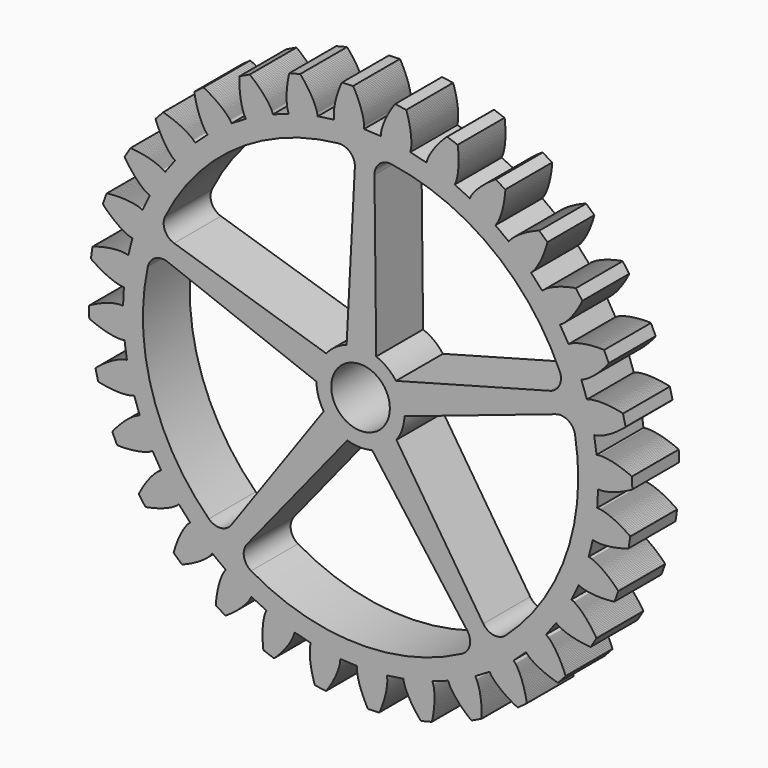
from build123d import *

# Parameters (mm, degrees)
F0_R     = 4
F1_DEPTH = 8


# Not quite as in the source:
# - ends of sketch curves that miss each other by under 0.0002 mm in the source are joined


with BuildPart() as f1:
    # F0 (on Front) → F1 (new body)
    with BuildSketch(Plane.XZ):
        Polygon((-32.30495, 2.758791), (-32.418904, 0.483381), (-32.827953, 0.489421), (-32.836156, 0.489353), (-32.848265, 0.489121), (-32.864272, 0.488639), (-32.884176, 0.487826), (-32.90797, 0.486592), (-32.93565, 0.484856), (-32.967203, 0.482529), (-33.002622, 0.47953), (-33.041894, 0.475776), (-33.085007, 0.471178), (-33.131944, 0.465651), (-33.182695, 0.459117), (-33.237238, 0.45149), (-33.29556, 0.442681), (-33.357637, 0.432614), (-33.423449, 0.421205), (-33.492973, 0.408367), (-33.566185, 0.394022), (-33.643063, 0.378087), (-33.723579, 0.36048), (-33.807704, 0.341119), (-33.89541, 0.319922), (-33.986665, 0.296816), (-34.081439, 0.271712), (-34.179699, 0.244537), (-34.281407, 0.215206), (-34.386532, 0.183647), (-34.495036, 0.149779), (-34.60688, 0.113524), (-34.722023, 0.07481), (-34.840427, 0.033554), (-34.962046, -0.010314), (-35.086841, -0.056873), (-35.214765, -0.106196), (-35.345772, -0.158355), (-35.479815, -0.213426), (-35.616844, -0.271479), (-35.756814, -0.332584), (-35.899674, -0.396816), (-36.045365, -0.464242), (-36.19384, -0.534931), (-36.345044, -0.608957), (-36.498922, -0.686378), (-36.655413, -0.767272), (-36.814466, -0.851694), (-36.976019, -0.939718), (-37.102372, -1.03036), (-37.029669, -2.539949), (-36.895187, -2.618028), (-36.725926, -2.69012), (-36.559495, -2.758869), (-36.395953, -2.824345), (-36.235347, -2.886624), (-36.077731, -2.945775), (-35.923148, -3.001868), (-35.771652, -3.05498), (-35.623283, -3.105186), (-35.478088, -3.152558), (-35.336111, -3.197173), (-35.197396, -3.239109), (-35.061983, -3.278438), (-34.929912, -3.315237), (-34.801221, -3.349589), (-34.67595, -3.381567), (-34.55413, -3.411253), (-34.435797, -3.438723), (-34.320987, -3.464063), (-34.209733, -3.487346), (-34.102062, -3.508656), (-33.998002, -3.528075), (-33.897586, -3.545683), (-33.800839, -3.56156), (-33.707785, -3.575794), (-33.618449, -3.588462), (-33.532853, -3.599649), (-33.45102, -3.609438), (-33.372967, -3.617912), (-33.298711, -3.625154), (-33.228277, -3.631252), (-33.161672, -3.636284), (-33.098917, -3.640337), (-33.040018, -3.643499), (-32.984994, -3.645852), (-32.93385, -3.647479), (-32.886599, -3.648479), (-32.843243, -3.648928), (-32.80379, -3.648891), (-32.76825, -3.648471), (-32.736619, -3.647754), (-32.708902, -3.646824), (-32.685097, -3.645764), (-32.665206, -3.644662), (-32.649229, -3.643603), (-32.637155, -3.64267), (-32.628982, -3.64195), (-32.222407, -3.596628), (-31.890287, -5.850547), (-32.292656, -5.924424), (-32.30069, -5.926093), (-32.312516, -5.928684), (-32.328121, -5.932277), (-32.347486, -5.93696), (-32.370583, -5.94281), (-32.39739, -5.949914), (-32.427885, -5.958352), (-32.462036, -5.968202), (-32.499823, -5.979548), (-32.54121, -5.992468), (-32.586169, -6.007045), (-32.634668, -6.023353), (-32.686676, -6.041477), (-32.742158, -6.061491), (-32.801078, -6.083474), (-32.8634, -6.107507), (-32.929084, -6.13366), (-32.998093, -6.162015), (-33.070382, -6.192642), (-33.145916, -6.225619), (-33.224646, -6.261018), (-33.306532, -6.298915), (-33.391525, -6.339385), (-33.479581, -6.382493), (-33.570651, -6.428317), (-33.664684, -6.476926), (-33.761633, -6.528388), (-33.861445, -6.582774), (-33.964066, -6.640148), (-34.069445, -6.700586), (-34.177523, -6.764147), (-34.288249, -6.830899), (-34.40156, -6.900911), (-34.517406, -6.974242), (-34.635719, -7.050959), (-34.756442, -7.131121), (-34.879514, -7.21479), (-35.004876, -7.30203), (-35.132456, -7.392896), (-35.262195, -7.48745), (-35.394027, -7.585747), (-35.527884, -7.687849), (-35.663698, -7.793802), (-35.801404, -7.903672), (-35.940929, -8.017503), (-36.082204, -8.13535), (-36.188447, -8.248902), (-35.822632, -9.7153), (-35.675507, -9.765645), (-35.495432, -9.803327), (-35.318789, -9.838286), (-35.145615, -9.870601), (-34.975945, -9.90035), (-34.809816, -9.927615), (-34.64726, -9.952475), (-34.488312, -9.975011), (-34.332999, -9.995305), (-34.181354, -10.013442), (-34.0334, -10.0295), (-33.889169, -10.043566), (-33.748687, -10.055723), (-33.611973, -10.066051), (-33.479056, -10.074633), (-33.349949, -10.081559), (-33.224681, -10.086909), (-33.103262, -10.090766), (-32.985716, -10.09322), (-32.872055, -10.094351), (-32.762296, -10.094245), (-32.656447, -10.09299), (-32.554525, -10.090671), (-32.456539, -10.08737), (-32.362497, -10.083175), (-32.272405, -10.07817), (-32.186273, -10.072442), (-32.1041, -10.066078), (-32.025893, -10.059164), (-31.951655, -10.051781), (-31.881384, -10.044018), (-31.815079, -10.03596), (-31.752737, -10.027696), (-31.694353, -10.019304), (-31.639928, -10.010875), (-31.589447, -10.002496), (-31.542909, -9.994245), (-31.500305, -9.986214), (-31.461619, -9.978481), (-31.426839, -9.971136), (-31.395958, -9.964262), (-31.368954, -9.957941), (-31.345814, -9.952259), (-31.32652, -9.947296), (-31.311054, -9.943141), (-31.299397, -9.939873), (-31.291522, -9.937573), (-30.901601, -9.8138), (-30.136143, -11.959618), (-30.516371, -12.110574), (-30.523923, -12.113776), (-30.535017, -12.118625), (-30.549621, -12.125193), (-30.567698, -12.133564), (-30.589213, -12.14381), (-30.614117, -12.156006), (-30.64238, -12.170229), (-30.673955, -12.186554), (-30.708799, -12.205051), (-30.74687, -12.2258), (-30.788123, -12.248866), (-30.832511, -12.274325), (-30.879984, -12.302247), (-30.930496, -12.332701), (-30.983994, -12.365758), (-31.040427, -12.401483), (-31.099748, -12.439948), (-31.161897, -12.481222), (-31.226825, -12.525362), (-31.294475, -12.572442), (-31.364787, -12.622522), (-31.437703, -12.675668), (-31.513172, -12.731937), (-31.591124, -12.791399), (-31.671503, -12.854109), (-31.754247, -12.920128), (-31.839292, -12.989513), (-31.926575, -13.062327), (-32.016033, -13.138622), (-32.107594, -13.218453), (-32.201197, -13.30188), (-32.296773, -13.388952), (-32.394248, -13.479723), (-32.493562, -13.574246), (-32.594635, -13.672569), (-32.6974, -13.774741), (-32.801785, -13.880817), (-32.907717, -13.990836), (-33.015119, -14.104845), (-33.123918, -14.222894), (-33.234039, -14.345022), (-33.345407, -14.471274), (-33.457941, -14.601692), (-33.571567, -14.736312), (-33.686202, -14.875178), (-33.801772, -15.018324), (-33.883821, -15.150418), (-33.238955, -16.517272), (-33.084833, -16.537945), (-32.900866, -16.539774), (-32.720798, -16.539603), (-32.544647, -16.53751), (-32.372435, -16.533586), (-32.20418, -16.527916), (-32.039896, -16.520585), (-31.879605, -16.511678), (-31.72332, -16.501284), (-31.571049, -16.489487), (-31.422807, -16.476375), (-31.278602, -16.462033), (-31.138447, -16.446548), (-31.002345, -16.430006), (-30.870306, -16.412493), (-30.742332, -16.394097), (-30.618423, -16.374903), (-30.498586, -16.355001), (-30.38282, -16.334474), (-30.271124, -16.313412), (-30.163492, -16.291896), (-30.059923, -16.270015), (-29.960415, -16.247854), (-29.864955, -16.225501), (-29.773535, -16.203039), (-29.686154, -16.180556), (-29.602792, -16.158135), (-29.523439, -16.135863), (-29.448085, -16.11382), (-29.376712, -16.092097), (-29.309304, -16.070774), (-29.245845, -16.049936), (-29.186314, -16.029668), (-29.130691, -16.010049), (-29.078953, -15.991165), (-29.03108, -15.973095), (-28.987048, -15.955927), (-28.946828, -15.939737), (-28.910393, -15.924605), (-28.877716, -15.910618), (-28.848768, -15.89785), (-28.823514, -15.886383), (-28.80193, -15.876295), (-28.783973, -15.867664), (-28.769616, -15.860571), (-28.758821, -15.855088), (-28.751545, -15.851299), (-28.393263, -15.653834), (-27.223886, -17.609087), (-27.567356, -17.831322), (-27.574136, -17.835937), (-27.584075, -17.842854), (-27.597118, -17.852148), (-27.613215, -17.863883), (-27.632313, -17.878128), (-27.654361, -17.894952), (-27.679305, -17.914416), (-27.70709, -17.936585), (-27.737657, -17.961527), (-27.77095, -17.989303), (-27.806909, -18.019975), (-27.845476, -18.053601), (-27.886588, -18.090248), (-27.930189, -18.129971), (-27.976209, -18.17283), (-28.024591, -18.218881), (-28.075266, -18.26818), (-28.128171, -18.320783), (-28.183239, -18.376743), (-28.240401, -18.436115), (-28.299594, -18.498951), (-28.360742, -18.565299), (-28.42378, -18.635212), (-28.488635, -18.70874), (-28.555237, -18.785927), (-28.62351, -18.866819), (-28.693388, -18.951464), (-28.764789, -19.039905), (-28.83764, -19.132186), (-28.911869, -19.228348), (-28.987398, -19.328431), (-29.064148, -19.432475), (-29.142046, -19.54052), (-29.221006, -19.652599), (-29.300956, -19.768753), (-29.381814, -19.889011), (-29.463499, -20.01341), (-29.545931, -20.141983), (-29.629028, -20.274756), (-29.712707, -20.411761), (-29.796887, -20.553027), (-29.881482, -20.698581), (-29.966413, -20.848443), (-30.051592, -21.002645), (-30.136934, -21.161207), (-30.222355, -21.32415), (-30.277059, -21.469714), (-29.377922, -22.684498), (-29.22273, -22.674706), (-29.041943, -22.64061), (-28.865365, -22.60531), (-28.693007, -22.568894), (-28.524871, -22.531448), (-28.360953, -22.493061), (-28.20126, -22.453822), (-28.045785, -22.413816), (-27.894528, -22.373128), (-27.747484, -22.331853), (-27.604648, -22.29007), (-27.466014, -22.247871), (-27.331572, -22.20534), (-27.201315, -22.162564), (-27.075228, -22.11963), (-26.9533, -22.076622), (-26.835519, -22.033623), (-26.721866, -21.990724), (-26.61233, -21.948009), (-26.506888, -21.905557), (-26.405523, -21.863457), (-26.308213, -21.82179), (-26.21494, -21.780644), (-26.125674, -21.740096), (-26.040395, -21.700233), (-25.959078, -21.661132), (-25.88169, -21.62288), (-25.808211, -21.585555), (-25.738602, -21.549234), (-25.672841, -21.514006), (-25.610887, -21.479942), (-25.552712, -21.447122), (-25.498278, -21.415629), (-25.447552, -21.385538), (-25.400494, -21.356922), (-25.357066, -21.32986), (-25.317228, -21.304431), (-25.280937, -21.280705), (-25.248154, -21.258758), (-25.218835, -21.238662), (-25.192934, -21.220493), (-25.170404, -21.204318), (-25.151203, -21.190215), (-25.135277, -21.178245), (-25.122577, -21.168488), (-25.113059, -21.161004), (-25.106664, -21.155869), (-24.793788, -20.892301), (-23.265429, -22.581851), (-23.558942, -22.866824), (-23.564695, -22.872669), (-23.573089, -22.881398), (-23.584069, -22.893055), (-23.597569, -22.907707), (-23.613521, -22.925402), (-23.631866, -22.946202), (-23.652534, -22.970158), (-23.675457, -22.997323), (-23.700571, -23.02775), (-23.727804, -23.061486), (-23.757089, -23.098585), (-23.788353, -23.13909), (-23.82153, -23.183052), (-23.85654, -23.230518), (-23.893317, -23.281533), (-23.931785, -23.336137), (-23.971869, -23.394374), (-24.013495, -23.456287), (-24.056588, -23.521918), (-24.101067, -23.591302), (-24.146864, -23.664475), (-24.193893, -23.741479), (-24.242081, -23.822346), (-24.291345, -23.907112), (-24.341608, -23.995809), (-24.392792, -24.088466), (-24.444808, -24.18512), (-24.497585, -24.28579), (-24.551034, -24.390509), (-24.605076, -24.499307), (-24.65963, -24.612201), (-24.714606, -24.729219), (-24.769929, -24.850385), (-24.825507, -24.975717), (-24.881259, -25.105235), (-24.937103, -25.238958), (-24.992948, -25.376903), (-25.048715, -25.519087), (-25.10431, -25.665518), (-25.159654, -25.816218), (-25.214655, -25.97119), (-25.269233, -26.13045), (-25.323291, -26.294005), (-25.376749, -26.46186), (-25.429521, -26.634026), (-25.481512, -26.8105), (-25.506763, -26.963938), (-24.387916, -27.97997), (-24.237611, -27.94009), (-24.066949, -27.871379), (-23.900654, -27.802308), (-23.738711, -27.732966), (-23.581112, -27.663438), (-23.427831, -27.59381), (-23.278861, -27.52417), (-23.134179, -27.4546), (-22.993768, -27.385189), (-22.857601, -27.316019), (-22.725662, -27.247173), (-22.597924, -27.178739), (-22.474363, -27.110797), (-22.354951, -27.043431), (-22.239666, -26.976721), (-22.12847, -26.910753), (-22.02134, -26.845605), (-21.918243, -26.781356), (-21.819144, -26.71809), (-21.724007, -26.655884), (-21.632804, -26.594819), (-21.545495, -26.53497), (-21.462037, -26.476416), (-21.382399, -26.419233), (-21.306535, -26.363497), (-21.234409, -26.309284), (-21.165972, -26.256671), (-21.101186, -26.205725), (-21.040002, -26.156525), (-20.982376, -26.109144), (-20.928257, -26.063647), (-20.877603, -26.02011), (-20.830359, -25.978601), (-20.786478, -25.939191), (-20.745907, -25.901946), (-20.708593, -25.866932), (-20.67448, -25.834219), (-20.643518, -25.803869), (-20.615647, -25.775946), (-20.590811, -25.75052), (-20.568951, -25.727643), (-20.550012, -25.707386), (-20.533927, -25.689808), (-20.520643, -25.674962), (-20.510094, -25.662915), (-20.502214, -25.653717), (-20.496945, -25.647432), (-20.2415, -25.32789), (-18.412894, -26.686808), (-18.645173, -27.023566), (-18.649674, -27.030423), (-18.656207, -27.04062), (-18.664699, -27.054194), (-18.67508, -27.071199), (-18.687275, -27.091669), (-18.701209, -27.115646), (-18.716804, -27.143176), (-18.733988, -27.174291), (-18.752685, -27.209029), (-18.772815, -27.24743), (-18.7943, -27.289529), (-18.817059, -27.335356), (-18.841021, -27.384948), (-18.8661, -27.438333), (-18.892216, -27.495541), (-18.919294, -27.556599), (-18.947244, -27.621539), (-18.975994, -27.690385), (-19.005453, -27.763159), (-19.035545, -27.839885), (-19.066184, -27.920588), (-19.097289, -28.005287), (-19.128771, -28.094003), (-19.160552, -28.186752), (-19.192545, -28.28355), (-19.224667, -28.384411), (-19.25683, -28.489353), (-19.288953, -28.598389), (-19.320947, -28.711524), (-19.352724, -28.82877), (-19.384205, -28.950141), (-19.415295, -29.075635), (-19.445914, -29.205266), (-19.475975, -29.339033), (-19.505391, -29.476939), (-19.534072, -29.618986), (-19.561934, -29.765176), (-19.588888, -29.915507), (-19.614849, -30.069972), (-19.639728, -30.228571), (-19.663441, -30.391298), (-19.685896, -30.558144), (-19.70701, -30.729102), (-19.726694, -30.904161), (-19.744865, -31.083312), (-19.761428, -31.266541), (-19.756262, -31.421959), (-18.46069, -32.200188), (-18.321056, -32.131751), (-18.16708, -32.031066), (-18.017455, -31.93088), (-17.872152, -31.831278), (-17.731143, -31.732338), (-17.594393, -31.634148), (-17.461871, -31.536782), (-17.333542, -31.440323), (-17.209367, -31.344851), (-17.089313, -31.250447), (-16.97334, -31.157184), (-16.861408, -31.065144), (-16.753475, -30.974402), (-16.649502, -30.885034), (-16.549442, -30.797115), (-16.453257, -30.710721), (-16.360895, -30.625923), (-16.272311, -30.542798), (-16.187458, -30.461413), (-16.106287, -30.381843), (-16.02875, -30.304158), (-15.954794, -30.228427), (-15.884365, -30.154717), (-15.81741, -30.083094), (-15.75388, -30.01363), (-15.693714, -29.946387), (-15.636858, -29.881433), (-15.583254, -29.818827), (-15.532843, -29.758637), (-15.485567, -29.700923), (-15.441368, -29.645744), (-15.400179, -29.593159), (-15.361942, -29.543233), (-15.326591, -29.496018), (-15.294066, -29.451572), (-15.264301, -29.409954), (-15.237226, -29.371213), (-15.212778, -29.335405), (-15.190891, -29.302584), (-15.171492, -29.272796), (-15.154514, -29.246099), (-15.139892, -29.222535), (-15.127548, -29.202156), (-15.117414, -29.185004), (-15.109415, -29.171127), (-15.103483, -29.160574), (-15.099544, -29.153378), (-14.911346, -28.790142), (-12.852764, -29.766205), (-13.014881, -30.141808), (-13.017955, -30.149413), (-13.022375, -30.160687), (-13.028058, -30.175659), (-13.03492, -30.19436), (-13.042887, -30.216815), (-13.051876, -30.243051), (-13.061802, -30.273096), (-13.072586, -30.306963), (-13.084143, -30.344683), (-13.096394, -30.386274), (-13.109254, -30.431754), (-13.122636, -30.481144), (-13.136464, -30.534454), (-13.150645, -30.591705), (-13.165101, -30.652909), (-13.179744, -30.718077), (-13.194489, -30.787223), (-13.209254, -30.860355), (-13.223951, -30.937477), (-13.238495, -31.0186), (-13.2528, -31.103733), (-13.266782, -31.19287), (-13.280355, -31.286025), (-13.293431, -31.383191), (-13.305926, -31.48437), (-13.317752, -31.589562), (-13.328824, -31.698762), (-13.339057, -31.811966), (-13.348364, -31.929171), (-13.356659, -32.050363), (-13.363855, -32.175542), (-13.369865, -32.304692), (-13.374608, -32.437804), (-13.377994, -32.574867), (-13.379933, -32.715862), (-13.380351, -32.860774), (-13.379157, -33.009592), (-13.376265, -33.16229), (-13.371594, -33.318853), (-13.365054, -33.47926), (-13.356563, -33.643486), (-13.346038, -33.811505), (-13.333396, -33.9833), (-13.318549, -34.158835), (-13.301415, -34.338089), (-13.281916, -34.521027), (-13.246527, -34.672451), (-11.824027, -35.182975), (-11.700429, -35.08861), (-11.56905, -34.95982), (-11.441847, -34.832369), (-11.318766, -34.706334), (-11.199769, -34.581787), (-11.084804, -34.458802), (-10.973824, -34.337454), (-10.866776, -34.217812), (-10.763617, -34.09995), (-10.664284, -33.983937), (-10.568734, -33.869843), (-10.476908, -33.757734), (-10.388755, -33.647679), (-10.304213, -33.539743), (-10.223228, -33.433993), (-10.145746, -33.330494), (-10.071701, -33.229308), (-10.001035, -33.130496), (-9.933692, -33.034124), (-9.869605, -32.940248), (-9.808713, -32.848928), (-9.75095, -32.760221), (-9.696255, -32.674187), (-9.644563, -32.590879), (-9.595804, -32.510357), (-9.549911, -32.432669), (-9.506818, -32.35787), (-9.466459, -32.286011), (-9.428761, -32.217141), (-9.393653, -32.151313), (-9.361068, -32.088571), (-9.330927, -32.028963), (-9.303165, -31.972533), (-9.277708, -31.919331), (-9.254479, -31.869394), (-9.233401, -31.822766), (-9.214407, -31.77949), (-9.197416, -31.7396), (-9.182349, -31.703138), (-9.169135, -31.670142), (-9.157694, -31.640641), (-9.147945, -31.614679), (-9.139816, -31.592282), (-9.133221, -31.573485), (-9.128085, -31.558314), (-9.124327, -31.546805), (-9.121865, -31.538981), (-9.008148, -31.146008), (-6.798701, -31.701707), (-6.884427, -32.10172), (-6.885962, -32.109777), (-6.888095, -32.121697), (-6.890744, -32.137491), (-6.893828, -32.157172), (-6.897262, -32.180749), (-6.900957, -32.208237), (-6.904835, -32.239636), (-6.908804, -32.27496), (-6.912779, -32.314209), (-6.916682, -32.357392), (-6.920421, -32.404505), (-6.92391, -32.455555), (-6.927072, -32.51054), (-6.929811, -32.569459), (-6.932048, -32.632306), (-6.933696, -32.69908), (-6.934684, -32.769774), (-6.934896, -32.844377), (-6.934265, -32.922887), (-6.932703, -33.005289), (-6.930125, -33.091574), (-6.926448, -33.181731), (-6.921587, -33.275741), (-6.915457, -33.373592), (-6.907973, -33.475263), (-6.899051, -33.580741), (-6.888607, -33.690003), (-6.876556, -33.803029), (-6.862817, -33.919797), (-6.84731, -34.04028), (-6.829948, -34.164456), (-6.810646, -34.2923), (-6.789329, -34.423779), (-6.76591, -34.558867), (-6.74031, -34.697532), (-6.712451, -34.839744), (-6.682247, -34.985467), (-6.649622, -35.134668), (-6.614493, -35.287313), (-6.576788, -35.44336), (-6.536422, -35.602774), (-6.493318, -35.765511), (-6.447403, -35.931536), (-6.398595, -36.100805), (-6.346822, -36.273271), (-6.292007, -36.448888), (-6.227759, -36.5905), (-4.732991, -36.813699), (-4.630177, -36.697034), (-4.526451, -36.54509), (-4.426555, -36.395271), (-4.33043, -36.247646), (-4.238016, -36.102274), (-4.149253, -35.959226), (-4.064076, -35.818558), (-3.98243, -35.680333), (-3.904244, -35.544609), (-3.829454, -35.411447), (-3.757998, -35.280902), (-3.689811, -35.153033), (-3.624819, -35.027894), (-3.56296, -34.905541), (-3.504164, -34.786025), (-3.448359, -34.669396), (-3.395476, -34.555711), (-3.345449, -34.445012), (-3.298198, -34.337351), (-3.253659, -34.232775), (-3.211751, -34.131329), (-3.172403, -34.033059), (-3.135543, -33.938007), (-3.101097, -33.846218), (-3.068982, -33.757728), (-3.039132, -33.672581), (-3.011461, -33.590812), (-2.985895, -33.51246), (-2.962355, -33.437559), (-2.940766, -33.366147), (-2.921045, -33.298251), (-2.903116, -33.233909), (-2.886895, -33.17315), (-2.872306, -33.116003), (-2.859264, -33.062491), (-2.84769, -33.012649), (-2.837503, -32.966497), (-2.828616, -32.92406), (-2.820954, -32.885361), (-2.814433, -32.850418), (-2.808967, -32.819256), (-2.804471, -32.791889), (-2.800868, -32.768337), (-2.798068, -32.748612), (-2.79599, -32.732734), (-2.794547, -32.720712), (-2.793659, -32.712557), (-2.758791, -32.30495), (-0.483381, -32.418904), (-0.489421, -32.827953), (-0.489353, -32.836156), (-0.489121, -32.848265), (-0.488639, -32.864272), (-0.487826, -32.884176), (-0.486592, -32.90797), (-0.484856, -32.93565), (-0.482529, -32.967203), (-0.47953, -33.002622), (-0.475776, -33.041894), (-0.471178, -33.085007), (-0.465651, -33.131944), (-0.459117, -33.182695), (-0.45149, -33.237238), (-0.442681, -33.29556), (-0.432614, -33.357637), (-0.421205, -33.423449), (-0.408367, -33.492973), (-0.394022, -33.566185), (-0.378087, -33.643063), (-0.36048, -33.723579), (-0.341119, -33.807704), (-0.319922, -33.89541), (-0.296816, -33.986665), (-0.271712, -34.081439), (-0.244537, -34.179699), (-0.215206, -34.281407), (-0.183647, -34.386532), (-0.149779, -34.495036), (-0.113524, -34.60688), (-0.07481, -34.722023), (-0.033554, -34.840427), (0.010314, -34.962046), (0.056873, -35.086841), (0.106196, -35.214765), (0.158355, -35.345772), (0.213426, -35.479815), (0.271479, -35.616844), (0.332584, -35.756814), (0.396816, -35.899674), (0.464242, -36.045365), (0.534931, -36.19384), (0.608957, -36.345044), (0.686378, -36.498922), (0.767272, -36.655413), (0.851694, -36.814466), (0.939718, -36.976019), (1.03036, -37.102372), (2.539949, -37.029669), (2.618028, -36.895187), (2.69012, -36.725926), (2.758869, -36.559495), (2.824345, -36.395953), (2.886624, -36.235347), (2.945775, -36.077731), (3.001868, -35.923148), (3.05498, -35.771652), (3.105186, -35.623283), (3.152558, -35.478088), (3.197173, -35.336111), (3.239109, -35.197396), (3.278438, -35.061983), (3.315237, -34.929912), (3.349589, -34.801221), (3.381567, -34.67595), (3.411253, -34.55413), (3.438723, -34.435797), (3.464063, -34.320987), (3.487346, -34.209733), (3.508656, -34.102062), (3.528075, -33.998002), (3.545683, -33.897586), (3.56156, -33.800839), (3.575794, -33.707785), (3.588462, -33.618449), (3.599649, -33.532853), (3.609438, -33.45102), (3.617912, -33.372967), (3.625154, -33.298711), (3.631252, -33.228277), (3.636284, -33.161672), (3.640337, -33.098917), (3.643499, -33.040018), (3.645852, -32.984994), (3.647479, -32.93385), (3.648479, -32.886599), (3.648928, -32.843243), (3.648891, -32.80379), (3.648471, -32.76825), (3.647754, -32.736619), (3.646824, -32.708902), (3.645764, -32.685097), (3.644662, -32.665206), (3.643603, -32.649229), (3.64267, -32.637155), (3.64195, -32.628982), (3.596628, -32.222407), (5.850547, -31.890287), (5.924424, -32.292656), (5.926093, -32.30069), (5.928684, -32.312516), (5.932277, -32.328121), (5.93696, -32.347486), (5.94281, -32.370583), (5.949914, -32.39739), (5.958352, -32.427885), (5.968202, -32.462036), (5.979548, -32.499823), (5.992468, -32.54121), (6.007045, -32.586169), (6.023353, -32.634668), (6.041477, -32.686676), (6.061491, -32.742158), (6.083474, -32.801078), (6.107507, -32.8634), (6.13366, -32.929084), (6.162015, -32.998093), (6.192642, -33.070382), (6.225619, -33.145916), (6.261018, -33.224646), (6.298915, -33.306532), (6.339385, -33.391525), (6.382493, -33.479581), (6.428317, -33.570651), (6.476926, -33.664684), (6.528388, -33.761633), (6.582774, -33.861445), (6.640148, -33.964066), (6.700586, -34.069445), (6.764147, -34.177523), (6.830899, -34.288249), (6.900911, -34.40156), (6.974242, -34.517406), (7.050959, -34.635719), (7.131121, -34.756442), (7.21479, -34.879514), (7.30203, -35.004876), (7.392896, -35.132456), (7.48745, -35.262195), (7.585747, -35.394027), (7.687849, -35.527884), (7.793802, -35.663698), (7.903672, -35.801404), (8.017503, -35.940929), (8.13535, -36.082204), (8.248902, -36.188447), (9.7153, -35.822632), (9.765645, -35.675507), (9.803327, -35.495432), (9.838286, -35.318789), (9.870601, -35.145615), (9.90035, -34.975945), (9.927615, -34.809816), (9.952475, -34.64726), (9.975011, -34.488312), (9.995305, -34.332999), (10.013442, -34.181354), (10.0295, -34.0334), (10.043566, -33.889169), (10.055723, -33.748687), (10.066051, -33.611973), (10.074633, -33.479056), (10.081559, -33.349949), (10.086909, -33.224681), (10.090766, -33.103262), (10.09322, -32.985716), (10.094351, -32.872055), (10.094245, -32.762296), (10.09299, -32.656447), (10.090671, -32.554525), (10.08737, -32.456539), (10.083175, -32.362497), (10.07817, -32.272405), (10.072442, -32.186273), (10.066078, -32.1041), (10.059164, -32.025893), (10.051781, -31.951655), (10.044018, -31.881384), (10.03596, -31.815079), (10.027696, -31.752737), (10.019304, -31.694353), (10.010875, -31.639928), (10.002496, -31.589447), (9.994245, -31.542909), (9.986214, -31.500305), (9.978481, -31.461619), (9.971136, -31.426839), (9.964262, -31.395958), (9.957941, -31.368954), (9.952259, -31.345814), (9.947296, -31.32652), (9.943141, -31.311054), (9.939873, -31.299397), (9.937573, -31.291522), (9.8138, -30.901601), (11.959618, -30.136143), (12.110574, -30.516371), (12.113776, -30.523923), (12.118625, -30.535017), (12.125193, -30.549621), (12.133564, -30.567698), (12.14381, -30.589213), (12.156006, -30.614117), (12.170229, -30.64238), (12.186554, -30.673955), (12.205051, -30.708799), (12.2258, -30.74687), (12.248866, -30.788123), (12.274325, -30.832511), (12.302247, -30.879984), (12.332701, -30.930496), (12.365758, -30.983994), (12.401483, -31.040427), (12.439948, -31.099748), (12.481222, -31.161897), (12.525362, -31.226825), (12.572442, -31.294475), (12.622522, -31.364787), (12.675668, -31.437703), (12.731937, -31.513172), (12.791399, -31.591124), (12.854109, -31.671503), (12.920128, -31.754247), (12.989513, -31.839292), (13.062327, -31.926575), (13.138622, -32.016033), (13.218453, -32.107594), (13.30188, -32.201197), (13.388952, -32.296773), (13.479723, -32.394248), (13.574246, -32.493562), (13.672569, -32.594635), (13.774741, -32.6974), (13.880817, -32.801785), (13.990836, -32.907717), (14.104845, -33.015119), (14.222894, -33.123918), (14.345022, -33.234039), (14.471274, -33.345407), (14.601692, -33.457941), (14.736312, -33.571567), (14.875178, -33.686202), (15.018324, -33.801772), (15.150418, -33.883821), (16.517272, -33.238955), (16.537945, -33.084833), (16.539774, -32.900866), (16.539603, -32.720798), (16.53751, -32.544647), (16.533586, -32.372435), (16.527916, -32.20418), (16.520585, -32.039896), (16.511678, -31.879605), (16.501284, -31.72332), (16.489487, -31.571049), (16.476375, -31.422807), (16.462033, -31.278602), (16.446548, -31.138447), (16.430006, -31.002345), (16.412493, -30.870306), (16.394097, -30.742332), (16.374903, -30.618423), (16.355001, -30.498586), (16.334474, -30.38282), (16.313412, -30.271124), (16.291896, -30.163492), (16.270015, -30.059923), (16.247854, -29.960415), (16.225501, -29.864955), (16.203039, -29.773535), (16.180556, -29.686154), (16.158135, -29.602792), (16.135863, -29.523439), (16.11382, -29.448085), (16.092097, -29.376712), (16.070774, -29.309304), (16.049936, -29.245845), (16.029668, -29.186314), (16.010049, -29.130691), (15.991165, -29.078953), (15.973095, -29.03108), (15.955927, -28.987048), (15.939737, -28.946828), (15.924605, -28.910393), (15.910618, -28.877716), (15.89785, -28.848768), (15.886383, -28.823514), (15.876295, -28.80193), (15.867664, -28.783973), (15.860571, -28.769616), (15.855088, -28.758821), (15.851299, -28.751545), (15.653834, -28.393263), (17.609087, -27.223886), (17.831322, -27.567356), (17.835937, -27.574136), (17.842854, -27.584075), (17.852148, -27.597118), (17.863883, -27.613215), (17.878128, -27.632313), (17.894952, -27.654361), (17.914416, -27.679305), (17.936585, -27.70709), (17.961527, -27.737657), (17.989303, -27.77095), (18.019975, -27.806909), (18.053601, -27.845476), (18.090248, -27.886588), (18.129971, -27.930189), (18.17283, -27.976209), (18.218881, -28.024591), (18.26818, -28.075266), (18.320783, -28.128171), (18.376743, -28.183239), (18.436115, -28.240401), (18.498951, -28.299594), (18.565299, -28.360742), (18.635212, -28.42378), (18.70874, -28.488635), (18.785927, -28.555237), (18.866819, -28.62351), (18.951464, -28.693388), (19.039905, -28.764789), (19.132186, -28.83764), (19.228348, -28.911869), (19.328431, -28.987398), (19.432475, -29.064148), (19.54052, -29.142046), (19.652599, -29.221006), (19.768753, -29.300956), (19.889011, -29.381814), (20.01341, -29.463499), (20.141983, -29.545931), (20.274756, -29.629028), (20.411761, -29.712707), (20.553027, -29.796887), (20.698581, -29.881482), (20.848443, -29.966413), (21.002645, -30.051592), (21.161207, -30.136934), (21.32415, -30.222355), (21.469714, -30.277059), (22.684498, -29.377922), (22.674706, -29.22273), (22.64061, -29.041943), (22.60531, -28.865365), (22.568894, -28.693007), (22.531448, -28.524871), (22.493061, -28.360953), (22.453822, -28.20126), (22.413816, -28.045785), (22.373128, -27.894528), (22.331853, -27.747484), (22.29007, -27.604648), (22.247871, -27.466014), (22.20534, -27.331572), (22.162564, -27.201315), (22.11963, -27.075228), (22.076622, -26.9533), (22.033623, -26.835519), (21.990724, -26.721866), (21.948009, -26.61233), (21.905557, -26.506888), (21.863457, -26.405523), (21.82179, -26.308213), (21.780644, -26.21494), (21.740096, -26.125674), (21.700233, -26.040395), (21.661132, -25.959078), (21.62288, -25.88169), (21.585555, -25.808211), (21.549234, -25.738602), (21.514006, -25.672841), (21.479942, -25.610887), (21.447122, -25.552712), (21.415629, -25.498278), (21.385538, -25.447552), (21.356922, -25.400494), (21.32986, -25.357066), (21.304431, -25.317228), (21.280705, -25.280937), (21.258758, -25.248154), (21.238662, -25.218835), (21.220493, -25.192934), (21.204318, -25.170404), (21.190215, -25.151203), (21.178245, -25.135277), (21.168488, -25.122577), (21.161004, -25.113059), (21.155869, -25.106664), (20.892301, -24.793788), (22.581851, -23.265429), (22.866824, -23.558942), (22.872669, -23.564695), (22.881398, -23.573089), (22.893055, -23.584069), (22.907707, -23.597569), (22.925402, -23.613521), (22.946202, -23.631866), (22.970158, -23.652534), (22.997323, -23.675457), (23.02775, -23.700571), (23.061486, -23.727804), (23.098585, -23.757089), (23.13909, -23.788353), (23.183052, -23.82153), (23.230518, -23.85654), (23.281533, -23.893317), (23.336137, -23.931785), (23.394374, -23.971869), (23.456287, -24.013495), (23.521918, -24.056588), (23.591302, -24.101067), (23.664475, -24.146864), (23.741479, -24.193893), (23.822346, -24.242081), (23.907112, -24.291345), (23.995809, -24.341608), (24.088466, -24.392792), (24.18512, -24.444808), (24.28579, -24.497585), (24.390509, -24.551034), (24.499307, -24.605076), (24.612201, -24.65963), (24.729219, -24.714606), (24.850385, -24.769929), (24.975717, -24.825507), (25.105235, -24.881259), (25.238958, -24.937103), (25.376903, -24.992948), (25.519087, -25.048715), (25.665518, -25.10431), (25.816218, -25.159654), (25.97119, -25.214655), (26.13045, -25.269233), (26.294005, -25.323291), (26.46186, -25.376749), (26.634026, -25.429521), (26.8105, -25.481512), (26.963938, -25.506763), (27.97997, -24.387916), (27.94009, -24.237611), (27.871379, -24.066949), (27.802308, -23.900654), (27.732966, -23.738711), (27.663438, -23.581112), (27.59381, -23.427831), (27.52417, -23.278861), (27.4546, -23.134179), (27.385189, -22.993768), (27.316019, -22.857601), (27.247173, -22.725662), (27.178739, -22.597924), (27.110797, -22.474363), (27.043431, -22.354951), (26.976721, -22.239666), (26.910753, -22.12847), (26.845605, -22.02134), (26.781356, -21.918243), (26.71809, -21.819144), (26.655884, -21.724007), (26.594819, -21.632804), (26.53497, -21.545495), (26.476416, -21.462037), (26.419233, -21.382399), (26.363497, -21.306535), (26.309284, -21.234409), (26.256671, -21.165972), (26.205725, -21.101186), (26.156525, -21.040002), (26.109144, -20.982376), (26.063647, -20.928257), (26.02011, -20.877603), (25.978601, -20.830359), (25.939191, -20.786478), (25.901946, -20.745907), (25.866932, -20.708593), (25.834219, -20.67448), (25.803869, -20.643518), (25.775946, -20.615647), (25.75052, -20.590811), (25.727643, -20.568951), (25.707386, -20.550012), (25.689808, -20.533927), (25.674962, -20.520643), (25.662915, -20.510094), (25.653717, -20.502214), (25.647432, -20.496945), (25.32789, -20.2415), (26.686808, -18.412894), (27.023566, -18.645173), (27.030423, -18.649674), (27.04062, -18.656207), (27.054194, -18.664699), (27.071199, -18.67508), (27.091669, -18.687275), (27.115646, -18.701209), (27.143176, -18.716804), (27.174291, -18.733988), (27.209029, -18.752685), (27.24743, -18.772815), (27.289529, -18.7943), (27.335356, -18.817059), (27.384948, -18.841021), (27.438333, -18.8661), (27.495541, -18.892216), (27.556599, -18.919294), (27.621539, -18.947244), (27.690385, -18.975994), (27.763159, -19.005453), (27.839885, -19.035545), (27.920588, -19.066184), (28.005287, -19.097289), (28.094003, -19.128771), (28.186752, -19.160552), (28.28355, -19.192545), (28.384411, -19.224667), (28.489353, -19.25683), (28.598389, -19.288953), (28.711524, -19.320947), (28.82877, -19.352724), (28.950141, -19.384205), (29.075635, -19.415295), (29.205266, -19.445914), (29.339033, -19.475975), (29.476939, -19.505391), (29.618986, -19.534072), (29.765176, -19.561934), (29.915507, -19.588888), (30.069972, -19.614849), (30.228571, -19.639728), (30.391298, -19.663441), (30.558144, -19.685896), (30.729102, -19.70701), (30.904161, -19.726694), (31.083312, -19.744865), (31.266541, -19.761428), (31.421959, -19.756262), (32.200188, -18.46069), (32.131751, -18.321056), (32.031066, -18.16708), (31.93088, -18.017455), (31.831278, -17.872152), (31.732338, -17.731143), (31.634148, -17.594393), (31.536782, -17.461871), (31.440323, -17.333542), (31.344851, -17.209367), (31.250447, -17.089313), (31.157184, -16.97334), (31.065144, -16.861408), (30.974402, -16.753475), (30.885034, -16.649502), (30.797115, -16.549442), (30.710721, -16.453257), (30.625923, -16.360895), (30.542798, -16.272311), (30.461413, -16.187458), (30.381843, -16.106287), (30.304158, -16.02875), (30.228427, -15.954794), (30.154717, -15.884365), (30.083094, -15.81741), (30.01363, -15.75388), (29.946387, -15.693714), (29.881433, -15.636858), (29.818827, -15.583254), (29.758637, -15.532843), (29.700923, -15.485567), (29.645744, -15.441368), (29.593159, -15.400179), (29.543233, -15.361942), (29.496018, -15.326591), (29.451572, -15.294066), (29.409954, -15.264301), (29.371213, -15.237226), (29.335405, -15.212778), (29.302584, -15.190891), (29.272796, -15.171492), (29.246099, -15.154514), (29.222535, -15.139892), (29.202156, -15.127548), (29.185004, -15.117414), (29.171127, -15.109415), (29.160574, -15.103483), (29.153378, -15.099544), (28.790142, -14.911346), (29.766205, -12.852764), (30.141808, -13.014881), (30.149413, -13.017955), (30.160687, -13.022375), (30.175659, -13.028058), (30.19436, -13.03492), (30.216815, -13.042887), (30.243051, -13.051876), (30.273096, -13.061802), (30.306963, -13.072586), (30.344683, -13.084143), (30.386274, -13.096394), (30.431754, -13.109254), (30.481144, -13.122636), (30.534454, -13.136464), (30.591705, -13.150645), (30.652909, -13.165101), (30.718077, -13.179744), (30.787223, -13.194489), (30.860355, -13.209254), (30.937477, -13.223951), (31.0186, -13.238495), (31.103733, -13.2528), (31.19287, -13.266782), (31.286025, -13.280355), (31.383191, -13.293431), (31.48437, -13.305926), (31.589562, -13.317752), (31.698762, -13.328824), (31.811966, -13.339057), (31.929171, -13.348364), (32.050363, -13.356659), (32.175542, -13.363855), (32.304692, -13.369865), (32.437804, -13.374608), (32.574867, -13.377994), (32.715862, -13.379933), (32.860774, -13.380351), (33.009592, -13.379157), (33.16229, -13.376265), (33.318853, -13.371594), (33.47926, -13.365054), (33.643486, -13.356563), (33.811505, -13.346038), (33.9833, -13.333396), (34.158835, -13.318549), (34.338089, -13.301415), (34.521027, -13.281916), (34.672451, -13.246527), (35.182975, -11.824027), (35.08861, -11.700429), (34.95982, -11.56905), (34.832369, -11.441847), (34.706334, -11.318766), (34.581787, -11.199769), (34.458802, -11.084804), (34.337454, -10.973824), (34.217812, -10.866776), (34.09995, -10.763617), (33.983937, -10.664284), (33.869843, -10.568734), (33.757734, -10.476908), (33.647679, -10.388755), (33.539743, -10.304213), (33.433993, -10.223228), (33.330494, -10.145746), (33.229308, -10.071701), (33.130496, -10.001035), (33.034124, -9.933692), (32.940248, -9.869605), (32.848928, -9.808713), (32.760221, -9.75095), (32.674187, -9.696255), (32.590879, -9.644563), (32.510357, -9.595804), (32.432669, -9.549911), (32.35787, -9.506818), (32.286011, -9.466459), (32.217141, -9.428761), (32.151313, -9.393653), (32.088571, -9.361068), (32.028963, -9.330927), (31.972533, -9.303165), (31.919331, -9.277708), (31.869394, -9.254479), (31.822766, -9.233401), (31.77949, -9.214407), (31.7396, -9.197416), (31.703138, -9.182349), (31.670142, -9.169135), (31.640641, -9.157694), (31.614679, -9.147945), (31.592282, -9.139816), (31.573485, -9.133221), (31.558314, -9.128085), (31.546805, -9.124327), (31.538981, -9.121865), (31.146008, -9.008148), (31.701707, -6.798701), (32.10172, -6.884427), (32.109777, -6.885962), (32.121697, -6.888095), (32.137491, -6.890744), (32.157172, -6.893828), (32.180749, -6.897262), (32.208237, -6.900957), (32.239636, -6.904835), (32.27496, -6.908804), (32.314209, -6.912779), (32.357392, -6.916682), (32.404505, -6.920421), (32.455555, -6.92391), (32.51054, -6.927072), (32.569459, -6.929811), (32.632306, -6.932048), (32.69908, -6.933696), (32.769774, -6.934684), (32.844377, -6.934896), (32.922887, -6.934265), (33.005289, -6.932703), (33.091574, -6.930125), (33.181731, -6.926448), (33.275741, -6.921587), (33.373592, -6.915457), (33.475263, -6.907973), (33.580741, -6.899051), (33.690003, -6.888607), (33.803029, -6.876556), (33.919797, -6.862817), (34.04028, -6.84731), (34.164456, -6.829948), (34.2923, -6.810646), (34.423779, -6.789329), (34.558867, -6.76591), (34.697532, -6.74031), (34.839744, -6.712451), (34.985467, -6.682247), (35.134668, -6.649622), (35.287313, -6.614493), (35.44336, -6.576788), (35.602774, -6.536422), (35.765511, -6.493318), (35.931536, -6.447403), (36.100805, -6.398595), (36.273271, -6.346822), (36.448888, -6.292007), (36.5905, -6.227759), (36.813699, -4.732991), (36.697034, -4.630177), (36.54509, -4.526451), (36.395271, -4.426555), (36.247646, -4.33043), (36.102274, -4.238016), (35.959226, -4.149253), (35.818558, -4.064076), (35.680333, -3.98243), (35.544609, -3.904244), (35.411447, -3.829454), (35.280902, -3.757998), (35.153033, -3.689811), (35.027894, -3.624819), (34.905541, -3.56296), (34.786025, -3.504164), (34.669396, -3.448359), (34.555711, -3.395476), (34.445012, -3.345449), (34.337351, -3.298198), (34.232775, -3.253659), (34.131329, -3.211751), (34.033059, -3.172403), (33.938007, -3.135543), (33.846218, -3.101097), (33.757728, -3.068982), (33.672581, -3.039132), (33.590812, -3.011461), (33.51246, -2.985895), (33.437559, -2.962355), (33.366147, -2.940766), (33.298251, -2.921045), (33.233909, -2.903116), (33.17315, -2.886895), (33.116003, -2.872306), (33.062491, -2.859264), (33.012649, -2.84769), (32.966497, -2.837503), (32.92406, -2.828616), (32.885361, -2.820954), (32.850418, -2.814433), (32.819256, -2.808967), (32.791889, -2.804471), (32.768337, -2.800868), (32.748612, -2.798068), (32.732734, -2.79599), (32.720712, -2.794547), (32.712557, -2.793659), (32.30495, -2.758791), (32.418904, -0.483381), (32.827953, -0.489421), (32.836156, -0.489353), (32.848265, -0.489121), (32.864272, -0.488639), (32.884176, -0.487826), (32.90797, -0.486592), (32.93565, -0.484856), (32.967203, -0.482529), (33.002622, -0.47953), (33.041894, -0.475776), (33.085007, -0.471178), (33.131944, -0.465651), (33.182695, -0.459117), (33.237238, -0.45149), (33.29556, -0.442681), (33.357637, -0.432614), (33.423449, -0.421205), (33.492973, -0.408367), (33.566185, -0.394022), (33.643063, -0.378087), (33.723579, -0.36048), (33.807704, -0.341119), (33.89541, -0.319922), (33.986665, -0.296816), (34.081439, -0.271712), (34.179699, -0.244537), (34.281407, -0.215206), (34.386532, -0.183647), (34.495036, -0.149779), (34.60688, -0.113524), (34.722023, -0.07481), (34.840427, -0.033554), (34.962046, 0.010314), (35.086841, 0.056873), (35.214765, 0.106196), (35.345772, 0.158355), (35.479815, 0.213426), (35.616844, 0.271479), (35.756814, 0.332584), (35.899674, 0.396816), (36.045365, 0.464242), (36.19384, 0.534931), (36.345044, 0.608957), (36.498922, 0.686378), (36.655413, 0.767272), (36.814466, 0.851694), (36.976019, 0.939718), (37.102372, 1.03036), (37.029669, 2.539949), (36.895187, 2.618028), (36.725926, 2.69012), (36.559495, 2.758869), (36.395953, 2.824345), (36.235347, 2.886624), (36.077731, 2.945775), (35.923148, 3.001868), (35.771652, 3.05498), (35.623283, 3.105186), (35.478088, 3.152558), (35.336111, 3.197173), (35.197396, 3.239109), (35.061983, 3.278438), (34.929912, 3.315237), (34.801221, 3.349589), (34.67595, 3.381567), (34.55413, 3.411253), (34.435797, 3.438723), (34.320987, 3.464063), (34.209733, 3.487346), (34.102062, 3.508656), (33.998002, 3.528075), (33.897586, 3.545683), (33.800839, 3.56156), (33.707785, 3.575794), (33.618449, 3.588462), (33.532853, 3.599649), (33.45102, 3.609438), (33.372967, 3.617912), (33.298711, 3.625154), (33.228277, 3.631252), (33.161672, 3.636284), (33.098917, 3.640337), (33.040018, 3.643499), (32.984994, 3.645852), (32.93385, 3.647479), (32.886599, 3.648479), (32.843243, 3.648928), (32.80379, 3.648891), (32.76825, 3.648471), (32.736619, 3.647754), (32.708902, 3.646824), (32.685097, 3.645764), (32.665206, 3.644662), (32.649229, 3.643603), (32.637155, 3.64267), (32.628982, 3.64195), (32.222407, 3.596628), (31.890287, 5.850547), (32.292656, 5.924424), (32.30069, 5.926093), (32.312516, 5.928684), (32.328121, 5.932277), (32.347486, 5.93696), (32.370583, 5.94281), (32.39739, 5.949914), (32.427885, 5.958352), (32.462036, 5.968202), (32.499823, 5.979548), (32.54121, 5.992468), (32.586169, 6.007045), (32.634668, 6.023353), (32.686676, 6.041477), (32.742158, 6.061491), (32.801078, 6.083474), (32.8634, 6.107507), (32.929084, 6.13366), (32.998093, 6.162015), (33.070382, 6.192642), (33.145916, 6.225619), (33.224646, 6.261018), (33.306532, 6.298915), (33.391525, 6.339385), (33.479581, 6.382493), (33.570651, 6.428317), (33.664684, 6.476926), (33.761633, 6.528388), (33.861445, 6.582774), (33.964066, 6.640148), (34.069445, 6.700586), (34.177523, 6.764147), (34.288249, 6.830899), (34.40156, 6.900911), (34.517406, 6.974242), (34.635719, 7.050959), (34.756442, 7.131121), (34.879514, 7.21479), (35.004876, 7.30203), (35.132456, 7.392896), (35.262195, 7.48745), (35.394027, 7.585747), (35.527884, 7.687849), (35.663698, 7.793802), (35.801404, 7.903672), (35.940929, 8.017503), (36.082204, 8.13535), (36.188447, 8.248902), (35.822632, 9.7153), (35.675507, 9.765645), (35.495432, 9.803327), (35.318789, 9.838286), (35.145615, 9.870601), (34.975945, 9.90035), (34.809816, 9.927615), (34.64726, 9.952475), (34.488312, 9.975011), (34.332999, 9.995305), (34.181354, 10.013442), (34.0334, 10.0295), (33.889169, 10.043566), (33.748687, 10.055723), (33.611973, 10.066051), (33.479056, 10.074633), (33.349949, 10.081559), (33.224681, 10.086909), (33.103262, 10.090766), (32.985716, 10.09322), (32.872055, 10.094351), (32.762296, 10.094245), (32.656447, 10.09299), (32.554525, 10.090671), (32.456539, 10.08737), (32.362497, 10.083175), (32.272405, 10.07817), (32.186273, 10.072442), (32.1041, 10.066078), (32.025893, 10.059164), (31.951655, 10.051781), (31.881384, 10.044018), (31.815079, 10.03596), (31.752737, 10.027696), (31.694353, 10.019304), (31.639928, 10.010875), (31.589447, 10.002496), (31.542909, 9.994245), (31.500305, 9.986214), (31.461619, 9.978481), (31.426839, 9.971136), (31.395958, 9.964262), (31.368954, 9.957941), (31.345814, 9.952259), (31.32652, 9.947296), (31.311054, 9.943141), (31.299397, 9.939873), (31.291522, 9.937573), (30.901601, 9.8138), (30.136143, 11.959618), (30.516371, 12.110574), (30.523923, 12.113776), (30.535017, 12.118625), (30.549621, 12.125193), (30.567698, 12.133564), (30.589213, 12.14381), (30.614117, 12.156006), (30.64238, 12.170229), (30.673955, 12.186554), (30.708799, 12.205051), (30.74687, 12.2258), (30.788123, 12.248866), (30.832511, 12.274325), (30.879984, 12.302247), (30.930496, 12.332701), (30.983994, 12.365758), (31.040427, 12.401483), (31.099748, 12.439948), (31.161897, 12.481222), (31.226825, 12.525362), (31.294475, 12.572442), (31.364787, 12.622522), (31.437703, 12.675668), (31.513172, 12.731937), (31.591124, 12.791399), (31.671503, 12.854109), (31.754247, 12.920128), (31.839292, 12.989513), (31.926575, 13.062327), (32.016033, 13.138622), (32.107594, 13.218453), (32.201197, 13.30188), (32.296773, 13.388952), (32.394248, 13.479723), (32.493562, 13.574246), (32.594635, 13.672569), (32.6974, 13.774741), (32.801785, 13.880817), (32.907717, 13.990836), (33.015119, 14.104845), (33.123918, 14.222894), (33.234039, 14.345022), (33.345407, 14.471274), (33.457941, 14.601692), (33.571567, 14.736312), (33.686202, 14.875178), (33.801772, 15.018324), (33.883821, 15.150418), (33.238955, 16.517272), (33.084833, 16.537945), (32.900866, 16.539774), (32.720798, 16.539603), (32.544647, 16.53751), (32.372435, 16.533586), (32.20418, 16.527916), (32.039896, 16.520585), (31.879605, 16.511678), (31.72332, 16.501284), (31.571049, 16.489487), (31.422807, 16.476375), (31.278602, 16.462033), (31.138447, 16.446548), (31.002345, 16.430006), (30.870306, 16.412493), (30.742332, 16.394097), (30.618423, 16.374903), (30.498586, 16.355001), (30.38282, 16.334474), (30.271124, 16.313412), (30.163492, 16.291896), (30.059923, 16.270015), (29.960415, 16.247854), (29.864955, 16.225501), (29.773535, 16.203039), (29.686154, 16.180556), (29.602792, 16.158135), (29.523439, 16.135863), (29.448085, 16.11382), (29.376712, 16.092097), (29.309304, 16.070774), (29.245845, 16.049936), (29.186314, 16.029668), (29.130691, 16.010049), (29.078953, 15.991165), (29.03108, 15.973095), (28.987048, 15.955927), (28.946828, 15.939737), (28.910393, 15.924605), (28.877716, 15.910618), (28.848768, 15.89785), (28.823514, 15.886383), (28.80193, 15.876295), (28.783973, 15.867664), (28.769616, 15.860571), (28.758821, 15.855088), (28.751545, 15.851299), (28.393263, 15.653834), (27.223886, 17.609087), (27.567356, 17.831322), (27.574136, 17.835937), (27.584075, 17.842854), (27.597118, 17.852148), (27.613215, 17.863883), (27.632313, 17.878128), (27.654361, 17.894952), (27.679305, 17.914416), (27.70709, 17.936585), (27.737657, 17.961527), (27.77095, 17.989303), (27.806909, 18.019975), (27.845476, 18.053601), (27.886588, 18.090248), (27.930189, 18.129971), (27.976209, 18.17283), (28.024591, 18.218881), (28.075266, 18.26818), (28.128171, 18.320783), (28.183239, 18.376743), (28.240401, 18.436115), (28.299594, 18.498951), (28.360742, 18.565299), (28.42378, 18.635212), (28.488635, 18.70874), (28.555237, 18.785927), (28.62351, 18.866819), (28.693388, 18.951464), (28.764789, 19.039905), (28.83764, 19.132186), (28.911869, 19.228348), (28.987398, 19.328431), (29.064148, 19.432475), (29.142046, 19.54052), (29.221006, 19.652599), (29.300956, 19.768753), (29.381814, 19.889011), (29.463499, 20.01341), (29.545931, 20.141983), (29.629028, 20.274756), (29.712707, 20.411761), (29.796887, 20.553027), (29.881482, 20.698581), (29.966413, 20.848443), (30.051592, 21.002645), (30.136934, 21.161207), (30.222355, 21.32415), (30.277059, 21.469714), (29.377922, 22.684498), (29.22273, 22.674706), (29.041943, 22.64061), (28.865365, 22.60531), (28.693007, 22.568894), (28.524871, 22.531448), (28.360953, 22.493061), (28.20126, 22.453822), (28.045785, 22.413816), (27.894528, 22.373128), (27.747484, 22.331853), (27.604648, 22.29007), (27.466014, 22.247871), (27.331572, 22.20534), (27.201315, 22.162564), (27.075228, 22.11963), (26.9533, 22.076622), (26.835519, 22.033623), (26.721866, 21.990724), (26.61233, 21.948009), (26.506888, 21.905557), (26.405523, 21.863457), (26.308213, 21.82179), (26.21494, 21.780644), (26.125674, 21.740096), (26.040395, 21.700233), (25.959078, 21.661132), (25.88169, 21.62288), (25.808211, 21.585555), (25.738602, 21.549234), (25.672841, 21.514006), (25.610887, 21.479942), (25.552712, 21.447122), (25.498278, 21.415629), (25.447552, 21.385538), (25.400494, 21.356922), (25.357066, 21.32986), (25.317228, 21.304431), (25.280937, 21.280705), (25.248154, 21.258758), (25.218835, 21.238662), (25.192934, 21.220493), (25.170404, 21.204318), (25.151203, 21.190215), (25.135277, 21.178245), (25.122577, 21.168488), (25.113059, 21.161004), (25.106664, 21.155869), (24.793788, 20.892301), (23.265429, 22.581851), (23.558942, 22.866824), (23.564695, 22.872669), (23.573089, 22.881398), (23.584069, 22.893055), (23.597569, 22.907707), (23.613521, 22.925402), (23.631866, 22.946202), (23.652534, 22.970158), (23.675457, 22.997323), (23.700571, 23.02775), (23.727804, 23.061486), (23.757089, 23.098585), (23.788353, 23.13909), (23.82153, 23.183052), (23.85654, 23.230518), (23.893317, 23.281533), (23.931785, 23.336137), (23.971869, 23.394374), (24.013495, 23.456287), (24.056588, 23.521918), (24.101067, 23.591302), (24.146864, 23.664475), (24.193893, 23.741479), (24.242081, 23.822346), (24.291345, 23.907112), (24.341608, 23.995809), (24.392792, 24.088466), (24.444808, 24.18512), (24.497585, 24.28579), (24.551034, 24.390509), (24.605076, 24.499307), (24.65963, 24.612201), (24.714606, 24.729219), (24.769929, 24.850385), (24.825507, 24.975717), (24.881259, 25.105235), (24.937103, 25.238958), (24.992948, 25.376903), (25.048715, 25.519087), (25.10431, 25.665518), (25.159654, 25.816218), (25.214655, 25.97119), (25.269233, 26.13045), (25.323291, 26.294005), (25.376749, 26.46186), (25.429521, 26.634026), (25.481512, 26.8105), (25.506763, 26.963938), (24.387916, 27.97997), (24.237611, 27.94009), (24.066949, 27.871379), (23.900654, 27.802308), (23.738711, 27.732966), (23.581112, 27.663438), (23.427831, 27.59381), (23.278861, 27.52417), (23.134179, 27.4546), (22.993768, 27.385189), (22.857601, 27.316019), (22.725662, 27.247173), (22.597924, 27.178739), (22.474363, 27.110797), (22.354951, 27.043431), (22.239666, 26.976721), (22.12847, 26.910753), (22.02134, 26.845605), (21.918243, 26.781356), (21.819144, 26.71809), (21.724007, 26.655884), (21.632804, 26.594819), (21.545495, 26.53497), (21.462037, 26.476416), (21.382399, 26.419233), (21.306535, 26.363497), (21.234409, 26.309284), (21.165972, 26.256671), (21.101186, 26.205725), (21.040002, 26.156525), (20.982376, 26.109144), (20.928257, 26.063647), (20.877603, 26.02011), (20.830359, 25.978601), (20.786478, 25.939191), (20.745907, 25.901946), (20.708593, 25.866932), (20.67448, 25.834219), (20.643518, 25.803869), (20.615647, 25.775946), (20.590811, 25.75052), (20.568951, 25.727643), (20.550012, 25.707386), (20.533927, 25.689808), (20.520643, 25.674962), (20.510094, 25.662915), (20.502214, 25.653717), (20.496945, 25.647432), (20.2415, 25.32789), (18.412894, 26.686808), (18.645173, 27.023566), (18.649674, 27.030423), (18.656207, 27.04062), (18.664699, 27.054194), (18.67508, 27.071199), (18.687275, 27.091669), (18.701209, 27.115646), (18.716804, 27.143176), (18.733988, 27.174291), (18.752685, 27.209029), (18.772815, 27.24743), (18.7943, 27.289529), (18.817059, 27.335356), (18.841021, 27.384948), (18.8661, 27.438333), (18.892216, 27.495541), (18.919294, 27.556599), (18.947244, 27.621539), (18.975994, 27.690385), (19.005453, 27.763159), (19.035545, 27.839885), (19.066184, 27.920588), (19.097289, 28.005287), (19.128771, 28.094003), (19.160552, 28.186752), (19.192545, 28.28355), (19.224667, 28.384411), (19.25683, 28.489353), (19.288953, 28.598389), (19.320947, 28.711524), (19.352724, 28.82877), (19.384205, 28.950141), (19.415295, 29.075635), (19.445914, 29.205266), (19.475975, 29.339033), (19.505391, 29.476939), (19.534072, 29.618986), (19.561934, 29.765176), (19.588888, 29.915507), (19.614849, 30.069972), (19.639728, 30.228571), (19.663441, 30.391298), (19.685896, 30.558144), (19.70701, 30.729102), (19.726694, 30.904161), (19.744865, 31.083312), (19.761428, 31.266541), (19.756262, 31.421959), (18.46069, 32.200188), (18.321056, 32.131751), (18.16708, 32.031066), (18.017455, 31.93088), (17.872152, 31.831278), (17.731143, 31.732338), (17.594393, 31.634148), (17.461871, 31.536782), (17.333542, 31.440323), (17.209367, 31.344851), (17.089313, 31.250447), (16.97334, 31.157184), (16.861408, 31.065144), (16.753475, 30.974402), (16.649502, 30.885034), (16.549442, 30.797115), (16.453257, 30.710721), (16.360895, 30.625923), (16.272311, 30.542798), (16.187458, 30.461413), (16.106287, 30.381843), (16.02875, 30.304158), (15.954794, 30.228427), (15.884365, 30.154717), (15.81741, 30.083094), (15.75388, 30.01363), (15.693714, 29.946387), (15.636858, 29.881433), (15.583254, 29.818827), (15.532843, 29.758637), (15.485567, 29.700923), (15.441368, 29.645744), (15.400179, 29.593159), (15.361942, 29.543233), (15.326591, 29.496018), (15.294066, 29.451572), (15.264301, 29.409954), (15.237226, 29.371213), (15.212778, 29.335405), (15.190891, 29.302584), (15.171492, 29.272796), (15.154514, 29.246099), (15.139892, 29.222535), (15.127548, 29.202156), (15.117414, 29.185004), (15.109415, 29.171127), (15.103483, 29.160574), (15.099544, 29.153378), (14.911346, 28.790142), (12.852764, 29.766205), (13.014881, 30.141808), (13.017955, 30.149413), (13.022375, 30.160687), (13.028058, 30.175659), (13.03492, 30.19436), (13.042887, 30.216815), (13.051876, 30.243051), (13.061802, 30.273096), (13.072586, 30.306963), (13.084143, 30.344683), (13.096394, 30.386274), (13.109254, 30.431754), (13.122636, 30.481144), (13.136464, 30.534454), (13.150645, 30.591705), (13.165101, 30.652909), (13.179744, 30.718077), (13.194489, 30.787223), (13.209254, 30.860355), (13.223951, 30.937477), (13.238495, 31.0186), (13.2528, 31.103733), (13.266782, 31.19287), (13.280355, 31.286025), (13.293431, 31.383191), (13.305926, 31.48437), (13.317752, 31.589562), (13.328824, 31.698762), (13.339057, 31.811966), (13.348364, 31.929171), (13.356659, 32.050363), (13.363855, 32.175542), (13.369865, 32.304692), (13.374608, 32.437804), (13.377994, 32.574867), (13.379933, 32.715862), (13.380351, 32.860774), (13.379157, 33.009592), (13.376265, 33.16229), (13.371594, 33.318853), (13.365054, 33.47926), (13.356563, 33.643486), (13.346038, 33.811505), (13.333396, 33.9833), (13.318549, 34.158835), (13.301415, 34.338089), (13.281916, 34.521027), (13.246527, 34.672451), (11.824027, 35.182975), (11.700429, 35.08861), (11.56905, 34.95982), (11.441847, 34.832369), (11.318766, 34.706334), (11.199769, 34.581787), (11.084804, 34.458802), (10.973824, 34.337454), (10.866776, 34.217812), (10.763617, 34.09995), (10.664284, 33.983937), (10.568734, 33.869843), (10.476908, 33.757734), (10.388755, 33.647679), (10.304213, 33.539743), (10.223228, 33.433993), (10.145746, 33.330494), (10.071701, 33.229308), (10.001035, 33.130496), (9.933692, 33.034124), (9.869605, 32.940248), (9.808713, 32.848928), (9.75095, 32.760221), (9.696255, 32.674187), (9.644563, 32.590879), (9.595804, 32.510357), (9.549911, 32.432669), (9.506818, 32.35787), (9.466459, 32.286011), (9.428761, 32.217141), (9.393653, 32.151313), (9.361068, 32.088571), (9.330927, 32.028963), (9.303165, 31.972533), (9.277708, 31.919331), (9.254479, 31.869394), (9.233401, 31.822766), (9.214407, 31.77949), (9.197416, 31.7396), (9.182349, 31.703138), (9.169135, 31.670142), (9.157694, 31.640641), (9.147945, 31.614679), (9.139816, 31.592282), (9.133221, 31.573485), (9.128085, 31.558314), (9.124327, 31.546805), (9.121865, 31.538981), (9.008148, 31.146008), (6.798701, 31.701707), (6.884427, 32.10172), (6.885962, 32.109777), (6.888095, 32.121697), (6.890744, 32.137491), (6.893828, 32.157172), (6.897262, 32.180749), (6.900957, 32.208237), (6.904835, 32.239636), (6.908804, 32.27496), (6.912779, 32.314209), (6.916682, 32.357392), (6.920421, 32.404505), (6.92391, 32.455555), (6.927072, 32.51054), (6.929811, 32.569459), (6.932048, 32.632306), (6.933696, 32.69908), (6.934684, 32.769774), (6.934896, 32.844377), (6.934265, 32.922887), (6.932703, 33.005289), (6.930125, 33.091574), (6.926448, 33.181731), (6.921587, 33.275741), (6.915457, 33.373592), (6.907973, 33.475263), (6.899051, 33.580741), (6.888607, 33.690003), (6.876556, 33.803029), (6.862817, 33.919797), (6.84731, 34.04028), (6.829948, 34.164456), (6.810646, 34.2923), (6.789329, 34.423779), (6.76591, 34.558867), (6.74031, 34.697532), (6.712451, 34.839744), (6.682247, 34.985467), (6.649622, 35.134668), (6.614493, 35.287313), (6.576788, 35.44336), (6.536422, 35.602774), (6.493318, 35.765511), (6.447403, 35.931536), (6.398595, 36.100805), (6.346822, 36.273271), (6.292007, 36.448888), (6.227759, 36.5905), (4.732991, 36.813699), (4.630177, 36.697034), (4.526451, 36.54509), (4.426555, 36.395271), (4.33043, 36.247646), (4.238016, 36.102274), (4.149253, 35.959226), (4.064076, 35.818558), (3.98243, 35.680333), (3.904244, 35.544609), (3.829454, 35.411447), (3.757998, 35.280902), (3.689811, 35.153033), (3.624819, 35.027894), (3.56296, 34.905541), (3.504164, 34.786025), (3.448359, 34.669396), (3.395476, 34.555711), (3.345449, 34.445012), (3.298198, 34.337351), (3.253659, 34.232775), (3.211751, 34.131329), (3.172403, 34.033059), (3.135543, 33.938007), (3.101097, 33.846218), (3.068982, 33.757728), (3.039132, 33.672581), (3.011461, 33.590812), (2.985895, 33.51246), (2.962355, 33.437559), (2.940766, 33.366147), (2.921045, 33.298251), (2.903116, 33.233909), (2.886895, 33.17315), (2.872306, 33.116003), (2.859264, 33.062491), (2.84769, 33.012649), (2.837503, 32.966497), (2.828616, 32.92406), (2.820954, 32.885361), (2.814433, 32.850418), (2.808967, 32.819256), (2.804471, 32.791889), (2.800868, 32.768337), (2.798068, 32.748612), (2.79599, 32.732734), (2.794547, 32.720712), (2.793659, 32.712557), (2.758791, 32.30495), (0.483381, 32.418904), (0.489421, 32.827953), (0.489353, 32.836156), (0.489121, 32.848265), (0.488639, 32.864272), (0.487826, 32.884176), (0.486592, 32.90797), (0.484856, 32.93565), (0.482529, 32.967203), (0.47953, 33.002622), (0.475776, 33.041894), (0.471178, 33.085007), (0.465651, 33.131944), (0.459117, 33.182695), (0.45149, 33.237238), (0.442681, 33.29556), (0.432614, 33.357637), (0.421205, 33.423449), (0.408367, 33.492973), (0.394022, 33.566185), (0.378087, 33.643063), (0.36048, 33.723579), (0.341119, 33.807704), (0.319922, 33.89541), (0.296816, 33.986665), (0.271712, 34.081439), (0.244537, 34.179699), (0.215206, 34.281407), (0.183647, 34.386532), (0.149779, 34.495036), (0.113524, 34.60688), (0.07481, 34.722023), (0.033554, 34.840427), (-0.010314, 34.962046), (-0.056873, 35.086841), (-0.106196, 35.214765), (-0.158355, 35.345772), (-0.213426, 35.479815), (-0.271479, 35.616844), (-0.332584, 35.756814), (-0.396816, 35.899674), (-0.464242, 36.045365), (-0.534931, 36.19384), (-0.608957, 36.345044), (-0.686378, 36.498922), (-0.767272, 36.655413), (-0.851694, 36.814466), (-0.939718, 36.976019), (-1.03036, 37.102372), (-2.539949, 37.029669), (-2.618028, 36.895187), (-2.69012, 36.725926), (-2.758869, 36.559495), (-2.824345, 36.395953), (-2.886624, 36.235347), (-2.945775, 36.077731), (-3.001868, 35.923148), (-3.05498, 35.771652), (-3.105186, 35.623283), (-3.152558, 35.478088), (-3.197173, 35.336111), (-3.239109, 35.197396), (-3.278438, 35.061983), (-3.315237, 34.929912), (-3.349589, 34.801221), (-3.381567, 34.67595), (-3.411253, 34.55413), (-3.438723, 34.435797), (-3.464063, 34.320987), (-3.487346, 34.209733), (-3.508656, 34.102062), (-3.528075, 33.998002), (-3.545683, 33.897586), (-3.56156, 33.800839), (-3.575794, 33.707785), (-3.588462, 33.618449), (-3.599649, 33.532853), (-3.609438, 33.45102), (-3.617912, 33.372967), (-3.625154, 33.298711), (-3.631252, 33.228277), (-3.636284, 33.161672), (-3.640337, 33.098917), (-3.643499, 33.040018), (-3.645852, 32.984994), (-3.647479, 32.93385), (-3.648479, 32.886599), (-3.648928, 32.843243), (-3.648891, 32.80379), (-3.648471, 32.76825), (-3.647754, 32.736619), (-3.646824, 32.708902), (-3.645764, 32.685097), (-3.644662, 32.665206), (-3.643603, 32.649229), (-3.64267, 32.637155), (-3.64195, 32.628982), (-3.596628, 32.222407), (-5.850547, 31.890287), (-5.924424, 32.292656), (-5.926093, 32.30069), (-5.928684, 32.312516), (-5.932277, 32.328121), (-5.93696, 32.347486), (-5.94281, 32.370583), (-5.949914, 32.39739), (-5.958352, 32.427885), (-5.968202, 32.462036), (-5.979548, 32.499823), (-5.992468, 32.54121), (-6.007045, 32.586169), (-6.023353, 32.634668), (-6.041477, 32.686676), (-6.061491, 32.742158), (-6.083474, 32.801078), (-6.107507, 32.8634), (-6.13366, 32.929084), (-6.162015, 32.998093), (-6.192642, 33.070382), (-6.225619, 33.145916), (-6.261018, 33.224646), (-6.298915, 33.306532), (-6.339385, 33.391525), (-6.382493, 33.479581), (-6.428317, 33.570651), (-6.476926, 33.664684), (-6.528388, 33.761633), (-6.582774, 33.861445), (-6.640148, 33.964066), (-6.700586, 34.069445), (-6.764147, 34.177523), (-6.830899, 34.288249), (-6.900911, 34.40156), (-6.974242, 34.517406), (-7.050959, 34.635719), (-7.131121, 34.756442), (-7.21479, 34.879514), (-7.30203, 35.004876), (-7.392896, 35.132456), (-7.48745, 35.262195), (-7.585747, 35.394027), (-7.687849, 35.527884), (-7.793802, 35.663698), (-7.903672, 35.801404), (-8.017503, 35.940929), (-8.13535, 36.082204), (-8.248902, 36.188447), (-9.7153, 35.822632), (-9.765645, 35.675507), (-9.803327, 35.495432), (-9.838286, 35.318789), (-9.870601, 35.145615), (-9.90035, 34.975945), (-9.927615, 34.809816), (-9.952475, 34.64726), (-9.975011, 34.488312), (-9.995305, 34.332999), (-10.013442, 34.181354), (-10.0295, 34.0334), (-10.043566, 33.889169), (-10.055723, 33.748687), (-10.066051, 33.611973), (-10.074633, 33.479056), (-10.081559, 33.349949), (-10.086909, 33.224681), (-10.090766, 33.103262), (-10.09322, 32.985716), (-10.094351, 32.872055), (-10.094245, 32.762296), (-10.09299, 32.656447), (-10.090671, 32.554525), (-10.08737, 32.456539), (-10.083175, 32.362497), (-10.07817, 32.272405), (-10.072442, 32.186273), (-10.066078, 32.1041), (-10.059164, 32.025893), (-10.051781, 31.951655), (-10.044018, 31.881384), (-10.03596, 31.815079), (-10.027696, 31.752737), (-10.019304, 31.694353), (-10.010875, 31.639928), (-10.002496, 31.589447), (-9.994245, 31.542909), (-9.986214, 31.500305), (-9.978481, 31.461619), (-9.971136, 31.426839), (-9.964262, 31.395958), (-9.957941, 31.368954), (-9.952259, 31.345814), (-9.947296, 31.32652), (-9.943141, 31.311054), (-9.939873, 31.299397), (-9.937573, 31.291522), (-9.8138, 30.901601), (-11.959618, 30.136143), (-12.110574, 30.516371), (-12.113776, 30.523923), (-12.118625, 30.535017), (-12.125193, 30.549621), (-12.133564, 30.567698), (-12.14381, 30.589213), (-12.156006, 30.614117), (-12.170229, 30.64238), (-12.186554, 30.673955), (-12.205051, 30.708799), (-12.2258, 30.74687), (-12.248866, 30.788123), (-12.274325, 30.832511), (-12.302247, 30.879984), (-12.332701, 30.930496), (-12.365758, 30.983994), (-12.401483, 31.040427), (-12.439948, 31.099748), (-12.481222, 31.161897), (-12.525362, 31.226825), (-12.572442, 31.294475), (-12.622522, 31.364787), (-12.675668, 31.437703), (-12.731937, 31.513172), (-12.791399, 31.591124), (-12.854109, 31.671503), (-12.920128, 31.754247), (-12.989513, 31.839292), (-13.062327, 31.926575), (-13.138622, 32.016033), (-13.218453, 32.107594), (-13.30188, 32.201197), (-13.388952, 32.296773), (-13.479723, 32.394248), (-13.574246, 32.493562), (-13.672569, 32.594635), (-13.774741, 32.6974), (-13.880817, 32.801785), (-13.990836, 32.907717), (-14.104845, 33.015119), (-14.222894, 33.123918), (-14.345022, 33.234039), (-14.471274, 33.345407), (-14.601692, 33.457941), (-14.736312, 33.571567), (-14.875178, 33.686202), (-15.018324, 33.801772), (-15.150418, 33.883821), (-16.517272, 33.238955), (-16.537945, 33.084833), (-16.539774, 32.900866), (-16.539603, 32.720798), (-16.53751, 32.544647), (-16.533586, 32.372435), (-16.527916, 32.20418), (-16.520585, 32.039896), (-16.511678, 31.879605), (-16.501284, 31.72332), (-16.489487, 31.571049), (-16.476375, 31.422807), (-16.462033, 31.278602), (-16.446548, 31.138447), (-16.430006, 31.002345), (-16.412493, 30.870306), (-16.394097, 30.742332), (-16.374903, 30.618423), (-16.355001, 30.498586), (-16.334474, 30.38282), (-16.313412, 30.271124), (-16.291896, 30.163492), (-16.270015, 30.059923), (-16.247854, 29.960415), (-16.225501, 29.864955), (-16.203039, 29.773535), (-16.180556, 29.686154), (-16.158135, 29.602792), (-16.135863, 29.523439), (-16.11382, 29.448085), (-16.092097, 29.376712), (-16.070774, 29.309304), (-16.049936, 29.245845), (-16.029668, 29.186314), (-16.010049, 29.130691), (-15.991165, 29.078953), (-15.973095, 29.03108), (-15.955927, 28.987048), (-15.939737, 28.946828), (-15.924605, 28.910393), (-15.910618, 28.877716), (-15.89785, 28.848768), (-15.886383, 28.823514), (-15.876295, 28.80193), (-15.867664, 28.783973), (-15.860571, 28.769616), (-15.855088, 28.758821), (-15.851299, 28.751545), (-15.653834, 28.393263), (-17.609087, 27.223886), (-17.831322, 27.567356), (-17.835937, 27.574136), (-17.842854, 27.584075), (-17.852148, 27.597118), (-17.863883, 27.613215), (-17.878128, 27.632313), (-17.894952, 27.654361), (-17.914416, 27.679305), (-17.936585, 27.70709), (-17.961527, 27.737657), (-17.989303, 27.77095), (-18.019975, 27.806909), (-18.053601, 27.845476), (-18.090248, 27.886588), (-18.129971, 27.930189), (-18.17283, 27.976209), (-18.218881, 28.024591), (-18.26818, 28.075266), (-18.320783, 28.128171), (-18.376743, 28.183239), (-18.436115, 28.240401), (-18.498951, 28.299594), (-18.565299, 28.360742), (-18.635212, 28.42378), (-18.70874, 28.488635), (-18.785927, 28.555237), (-18.866819, 28.62351), (-18.951464, 28.693388), (-19.039905, 28.764789), (-19.132186, 28.83764), (-19.228348, 28.911869), (-19.328431, 28.987398), (-19.432475, 29.064148), (-19.54052, 29.142046), (-19.652599, 29.221006), (-19.768753, 29.300956), (-19.889011, 29.381814), (-20.01341, 29.463499), (-20.141983, 29.545931), (-20.274756, 29.629028), (-20.411761, 29.712707), (-20.553027, 29.796887), (-20.698581, 29.881482), (-20.848443, 29.966413), (-21.002645, 30.051592), (-21.161207, 30.136934), (-21.32415, 30.222355), (-21.469714, 30.277059), (-22.684498, 29.377922), (-22.674706, 29.22273), (-22.64061, 29.041943), (-22.60531, 28.865365), (-22.568894, 28.693007), (-22.531448, 28.524871), (-22.493061, 28.360953), (-22.453822, 28.20126), (-22.413816, 28.045785), (-22.373128, 27.894528), (-22.331853, 27.747484), (-22.29007, 27.604648), (-22.247871, 27.466014), (-22.20534, 27.331572), (-22.162564, 27.201315), (-22.11963, 27.075228), (-22.076622, 26.9533), (-22.033623, 26.835519), (-21.990724, 26.721866), (-21.948009, 26.61233), (-21.905557, 26.506888), (-21.863457, 26.405523), (-21.82179, 26.308213), (-21.780644, 26.21494), (-21.740096, 26.125674), (-21.700233, 26.040395), (-21.661132, 25.959078), (-21.62288, 25.88169), (-21.585555, 25.808211), (-21.549234, 25.738602), (-21.514006, 25.672841), (-21.479942, 25.610887), (-21.447122, 25.552712), (-21.415629, 25.498278), (-21.385538, 25.447552), (-21.356922, 25.400494), (-21.32986, 25.357066), (-21.304431, 25.317228), (-21.280705, 25.280937), (-21.258758, 25.248154), (-21.238662, 25.218835), (-21.220493, 25.192934), (-21.204318, 25.170404), (-21.190215, 25.151203), (-21.178245, 25.135277), (-21.168488, 25.122577), (-21.161004, 25.113059), (-21.155869, 25.106664), (-20.892301, 24.793788), (-22.581851, 23.265429), (-22.866824, 23.558942), (-22.872669, 23.564695), (-22.881398, 23.573089), (-22.893055, 23.584069), (-22.907707, 23.597569), (-22.925402, 23.613521), (-22.946202, 23.631866), (-22.970158, 23.652534), (-22.997323, 23.675457), (-23.02775, 23.700571), (-23.061486, 23.727804), (-23.098585, 23.757089), (-23.13909, 23.788353), (-23.183052, 23.82153), (-23.230518, 23.85654), (-23.281533, 23.893317), (-23.336137, 23.931785), (-23.394374, 23.971869), (-23.456287, 24.013495), (-23.521918, 24.056588), (-23.591302, 24.101067), (-23.664475, 24.146864), (-23.741479, 24.193893), (-23.822346, 24.242081), (-23.907112, 24.291345), (-23.995809, 24.341608), (-24.088466, 24.392792), (-24.18512, 24.444808), (-24.28579, 24.497585), (-24.390509, 24.551034), (-24.499307, 24.605076), (-24.612201, 24.65963), (-24.729219, 24.714606), (-24.850385, 24.769929), (-24.975717, 24.825507), (-25.105235, 24.881259), (-25.238958, 24.937103), (-25.376903, 24.992948), (-25.519087, 25.048715), (-25.665518, 25.10431), (-25.816218, 25.159654), (-25.97119, 25.214655), (-26.13045, 25.269233), (-26.294005, 25.323291), (-26.46186, 25.376749), (-26.634026, 25.429521), (-26.8105, 25.481512), (-26.963938, 25.506763), (-27.97997, 24.387916), (-27.94009, 24.237611), (-27.871379, 24.066949), (-27.802308, 23.900654), (-27.732966, 23.738711), (-27.663438, 23.581112), (-27.59381, 23.427831), (-27.52417, 23.278861), (-27.4546, 23.134179), (-27.385189, 22.993768), (-27.316019, 22.857601), (-27.247173, 22.725662), (-27.178739, 22.597924), (-27.110797, 22.474363), (-27.043431, 22.354951), (-26.976721, 22.239666), (-26.910753, 22.12847), (-26.845605, 22.02134), (-26.781356, 21.918243), (-26.71809, 21.819144), (-26.655884, 21.724007), (-26.594819, 21.632804), (-26.53497, 21.545495), (-26.476416, 21.462037), (-26.419233, 21.382399), (-26.363497, 21.306535), (-26.309284, 21.234409), (-26.256671, 21.165972), (-26.205725, 21.101186), (-26.156525, 21.040002), (-26.109144, 20.982376), (-26.063647, 20.928257), (-26.02011, 20.877603), (-25.978601, 20.830359), (-25.939191, 20.786478), (-25.901946, 20.745907), (-25.866932, 20.708593), (-25.834219, 20.67448), (-25.803869, 20.643518), (-25.775946, 20.615647), (-25.75052, 20.590811), (-25.727643, 20.568951), (-25.707386, 20.550012), (-25.689808, 20.533927), (-25.674962, 20.520643), (-25.662915, 20.510094), (-25.653717, 20.502214), (-25.647432, 20.496945), (-25.32789, 20.2415), (-26.686808, 18.412894), (-27.023566, 18.645173), (-27.030423, 18.649674), (-27.04062, 18.656207), (-27.054194, 18.664699), (-27.071199, 18.67508), (-27.091669, 18.687275), (-27.115646, 18.701209), (-27.143176, 18.716804), (-27.174291, 18.733988), (-27.209029, 18.752685), (-27.24743, 18.772815), (-27.289529, 18.7943), (-27.335356, 18.817059), (-27.384948, 18.841021), (-27.438333, 18.8661), (-27.495541, 18.892216), (-27.556599, 18.919294), (-27.621539, 18.947244), (-27.690385, 18.975994), (-27.763159, 19.005453), (-27.839885, 19.035545), (-27.920588, 19.066184), (-28.005287, 19.097289), (-28.094003, 19.128771), (-28.186752, 19.160552), (-28.28355, 19.192545), (-28.384411, 19.224667), (-28.489353, 19.25683), (-28.598389, 19.288953), (-28.711524, 19.320947), (-28.82877, 19.352724), (-28.950141, 19.384205), (-29.075635, 19.415295), (-29.205266, 19.445914), (-29.339033, 19.475975), (-29.476939, 19.505391), (-29.618986, 19.534072), (-29.765176, 19.561934), (-29.915507, 19.588888), (-30.069972, 19.614849), (-30.228571, 19.639728), (-30.391298, 19.663441), (-30.558144, 19.685896), (-30.729102, 19.70701), (-30.904161, 19.726694), (-31.083312, 19.744865), (-31.266541, 19.761428), (-31.421959, 19.756262), (-32.200188, 18.46069), (-32.131751, 18.321056), (-32.031066, 18.16708), (-31.93088, 18.017455), (-31.831278, 17.872152), (-31.732338, 17.731143), (-31.634148, 17.594393), (-31.536782, 17.461871), (-31.440323, 17.333542), (-31.344851, 17.209367), (-31.250447, 17.089313), (-31.157184, 16.97334), (-31.065144, 16.861408), (-30.974402, 16.753475), (-30.885034, 16.649502), (-30.797115, 16.549442), (-30.710721, 16.453257), (-30.625923, 16.360895), (-30.542798, 16.272311), (-30.461413, 16.187458), (-30.381843, 16.106287), (-30.304158, 16.02875), (-30.228427, 15.954794), (-30.154717, 15.884365), (-30.083094, 15.81741), (-30.01363, 15.75388), (-29.946387, 15.693714), (-29.881433, 15.636858), (-29.818827, 15.583254), (-29.758637, 15.532843), (-29.700923, 15.485567), (-29.645744, 15.441368), (-29.593159, 15.400179), (-29.543233, 15.361942), (-29.496018, 15.326591), (-29.451572, 15.294066), (-29.409954, 15.264301), (-29.371213, 15.237226), (-29.335405, 15.212778), (-29.302584, 15.190891), (-29.272796, 15.171492), (-29.246099, 15.154514), (-29.222535, 15.139892), (-29.202156, 15.127548), (-29.185004, 15.117414), (-29.171127, 15.109415), (-29.160574, 15.103483), (-29.153378, 15.099544), (-28.790142, 14.911346), (-29.766205, 12.852764), (-30.141808, 13.014881), (-30.149413, 13.017955), (-30.160687, 13.022375), (-30.175659, 13.028058), (-30.19436, 13.03492), (-30.216815, 13.042887), (-30.243051, 13.051876), (-30.273096, 13.061802), (-30.306963, 13.072586), (-30.344683, 13.084143), (-30.386274, 13.096394), (-30.431754, 13.109254), (-30.481144, 13.122636), (-30.534454, 13.136464), (-30.591705, 13.150645), (-30.652909, 13.165101), (-30.718077, 13.179744), (-30.787223, 13.194489), (-30.860355, 13.209254), (-30.937477, 13.223951), (-31.0186, 13.238495), (-31.103733, 13.2528), (-31.19287, 13.266782), (-31.286025, 13.280355), (-31.383191, 13.293431), (-31.48437, 13.305926), (-31.589562, 13.317752), (-31.698762, 13.328824), (-31.811966, 13.339057), (-31.929171, 13.348364), (-32.050363, 13.356659), (-32.175542, 13.363855), (-32.304692, 13.369865), (-32.437804, 13.374608), (-32.574867, 13.377994), (-32.715862, 13.379933), (-32.860774, 13.380351), (-33.009592, 13.379157), (-33.16229, 13.376265), (-33.318853, 13.371594), (-33.47926, 13.365054), (-33.643486, 13.356563), (-33.811505, 13.346038), (-33.9833, 13.333396), (-34.158835, 13.318549), (-34.338089, 13.301415), (-34.521027, 13.281916), (-34.672451, 13.246527), (-35.182975, 11.824027), (-35.08861, 11.700429), (-34.95982, 11.56905), (-34.832369, 11.441847), (-34.706334, 11.318766), (-34.581787, 11.199769), (-34.458802, 11.084804), (-34.337454, 10.973824), (-34.217812, 10.866776), (-34.09995, 10.763617), (-33.983937, 10.664284), (-33.869843, 10.568734), (-33.757734, 10.476908), (-33.647679, 10.388755), (-33.539743, 10.304213), (-33.433993, 10.223228), (-33.330494, 10.145746), (-33.229308, 10.071701), (-33.130496, 10.001035), (-33.034124, 9.933692), (-32.940248, 9.869605), (-32.848928, 9.808713), (-32.760221, 9.75095), (-32.674187, 9.696255), (-32.590879, 9.644563), (-32.510357, 9.595804), (-32.432669, 9.549911), (-32.35787, 9.506818), (-32.286011, 9.466459), (-32.217141, 9.428761), (-32.151313, 9.393653), (-32.088571, 9.361068), (-32.028963, 9.330927), (-31.972533, 9.303165), (-31.919331, 9.277708), (-31.869394, 9.254479), (-31.822766, 9.233401), (-31.77949, 9.214407), (-31.7396, 9.197416), (-31.703138, 9.182349), (-31.670142, 9.169135), (-31.640641, 9.157694), (-31.614679, 9.147945), (-31.592282, 9.139816), (-31.573485, 9.133221), (-31.558314, 9.128085), (-31.546805, 9.124327), (-31.538981, 9.121865), (-31.146008, 9.008148), (-31.701707, 6.798701), (-32.10172, 6.884427), (-32.109777, 6.885962), (-32.121697, 6.888095), (-32.137491, 6.890744), (-32.157172, 6.893828), (-32.180749, 6.897262), (-32.208237, 6.900957), (-32.239636, 6.904835), (-32.27496, 6.908804), (-32.314209, 6.912779), (-32.357392, 6.916682), (-32.404505, 6.920421), (-32.455555, 6.92391), (-32.51054, 6.927072), (-32.569459, 6.929811), (-32.632306, 6.932048), (-32.69908, 6.933696), (-32.769774, 6.934684), (-32.844377, 6.934896), (-32.922887, 6.934265), (-33.005289, 6.932703), (-33.091574, 6.930125), (-33.181731, 6.926448), (-33.275741, 6.921587), (-33.373592, 6.915457), (-33.475263, 6.907973), (-33.580741, 6.899051), (-33.690003, 6.888607), (-33.803029, 6.876556), (-33.919797, 6.862817), (-34.04028, 6.84731), (-34.164456, 6.829948), (-34.2923, 6.810646), (-34.423779, 6.789329), (-34.558867, 6.76591), (-34.697532, 6.74031), (-34.839744, 6.712451), (-34.985467, 6.682247), (-35.134668, 6.649622), (-35.287313, 6.614493), (-35.44336, 6.576788), (-35.602774, 6.536422), (-35.765511, 6.493318), (-35.931536, 6.447403), (-36.100805, 6.398595), (-36.273271, 6.346822), (-36.448888, 6.292007), (-36.5905, 6.227759), (-36.813699, 4.732991), (-36.697034, 4.630177), (-36.54509, 4.526451), (-36.395271, 4.426555), (-36.247646, 4.33043), (-36.102274, 4.238016), (-35.959226, 4.149253), (-35.818558, 4.064076), (-35.680333, 3.98243), (-35.544609, 3.904244), (-35.411447, 3.829454), (-35.280902, 3.757998), (-35.153033, 3.689811), (-35.027894, 3.624819), (-34.905541, 3.56296), (-34.786025, 3.504164), (-34.669396, 3.448359), (-34.555711, 3.395476), (-34.445012, 3.345449), (-34.337351, 3.298198), (-34.232775, 3.253659), (-34.131329, 3.211751), (-34.033059, 3.172403), (-33.938007, 3.135543), (-33.846218, 3.101097), (-33.757728, 3.068982), (-33.672581, 3.039132), (-33.590812, 3.011461), (-33.51246, 2.985895), (-33.437559, 2.962355), (-33.366147, 2.940766), (-33.298251, 2.921045), (-33.233909, 2.903116), (-33.17315, 2.886895), (-33.116003, 2.872306), (-33.062491, 2.859264), (-33.012649, 2.84769), (-32.966497, 2.837503), (-32.92406, 2.828616), (-32.885361, 2.820954), (-32.850418, 2.814433), (-32.819256, 2.808967), (-32.791889, 2.804471), (-32.768337, 2.800868), (-32.748612, 2.798068), (-32.732734, 2.79599), (-32.720712, 2.794547), (-32.712557, 2.793659), align=None)
        with BuildLine():
            ThreePointArc((-14.9396714887, -25.6862551208), (-15.9159281388, -24.298199279), (-15.4975093578, -22.6536015195))
            Line((-15.4975093578, -22.6536015195), (-1.813382, -5.737863))
            ThreePointArc((-1.813382, -5.737863), (-0.1230841053, -6.0163350847), (1.5771890816, -5.8072293006))
            Line((1.5771890816, -5.8072293006), (14.55802, -23.268487))
            ThreePointArc((14.55802, -23.268487), (14.908825165, -24.9288227641), (13.876614021, -26.2757890398))
            ThreePointArc((13.876614021, -26.2757890398), (-0.6077913899, -29.7087214462), (-14.9396714887, -25.6862551208))
        make_face(mode=Mode.SUBTRACT)
        with BuildLine():
            ThreePointArc((-29.0456927661, 6.2709819495), (-28.0272529221, 7.6283907161), (-26.3338483204, 7.738659164))
            Line((-26.3338483204, 7.738659164), (-6.017398, -0.048468))
            ThreePointArc((-6.017398, -0.048468), (-5.7599098837, -1.7420894582), (-5.0356252549, -3.2945281667))
            Line((-5.0356252549, -3.2945281667), (-17.630971, -21.035858))
            ThreePointArc((-17.630971, -21.035858), (-19.1016390403, -21.8825649543), (-20.7016504018, -21.317109384))
            ThreePointArc((-20.7016504018, -21.317109384), (-28.4424908727, -8.6024562363), (-29.0456927661, 6.2709819495))
        make_face(mode=Mode.SUBTRACT)
        with BuildLine():
            ThreePointArc((19.8124683781, -22.1459613048), (18.190668428, -22.6455040275), (16.7558612397, -21.7393548442))
            Line((16.7558612397, -21.7393548442), (4.896667, -3.497726))
            ThreePointArc((4.896667, -3.497726), (5.68383961, -1.9762097149), (6.0103814763, -0.2945370233))
            Line((6.0103814763, -0.2945370233), (26.628322, 6.655142))
            ThreePointArc((26.628322, 6.655142), (28.3157997456, 6.4757053194), (29.2778700212, 5.0777790037))
            ThreePointArc((29.2778700212, 5.0777790037), (28.0668553302, -9.75854355), (19.8124683781, -22.1459613048))
        make_face(mode=Mode.SUBTRACT)
        with BuildLine():
            ThreePointArc((-3.0115539663, 29.5619356688), (-1.4058667122, 29.0128042098), (-0.7777043057, 27.4363560159))
            Line((-0.7777043057, 27.4363560159), (-1.905574, 5.707908))
            ThreePointArc((-1.905574, 5.707908), (-3.4367355091, 4.9396646231), (-4.6893761691, 3.771099136))
            Line((-4.6893761691, 3.771099136), (-25.454559, 10.267612))
            ThreePointArc((-25.454559, 10.267612), (-26.7142878892, 11.4046533235), (-26.6709379314, 13.1010909663))
            ThreePointArc((-26.6709379314, 13.1010909663), (-16.9706347709, 24.392111344), (-3.0115539663, 29.5619356688))
        make_face(mode=Mode.SUBTRACT)
        Circle(F0_R, mode=Mode.SUBTRACT)
        with BuildLine():
            Line((2.137431, 5.625195), (1.899188, 27.381591))
            ThreePointArc((1.899188, 27.381591), (2.5913017808, 28.9310285983), (4.2181049203, 29.4140284443))
            ThreePointArc((4.2181049203, 29.4140284443), (17.9540619091, 23.6776097042), (27.1844508104, 11.9992989163))
            ThreePointArc((27.1844508104, 11.9992989163), (27.1583800485, 10.3025080166), (25.8532007467, 9.2179409434))
            Line((25.8532007467, 9.2179409434), (4.839689, 3.57615))
            ThreePointArc((4.839689, 3.57615), (3.6358903215, 4.7949701896), (2.137431, 5.625195))
        make_face(mode=Mode.SUBTRACT)
    extrude(amount=F1_DEPTH)


solid = f1.part
